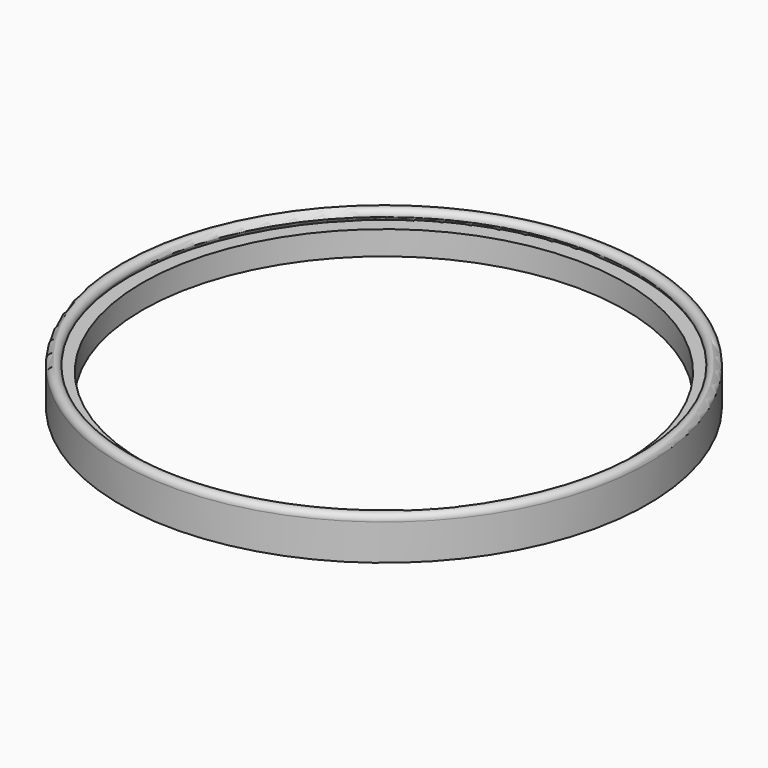
from build123d import *

# Parameters (mm, degrees)
F0_W = 8.2200646866
F0_H = 9.3895217869


# Not quite as in the source:
# - a feature names something its author has since deleted; it is built from what else it names


with BuildPart() as f1:
    # F0 (on Front) → F1 (revolve)
    with BuildSketch(Plane.XZ):
        with BuildLine():
            Line((0, 19), (0, 0))
            Line((0, 0), (0.6, 0))
            Line((0.6, 0), (0.6, 3.5557271383))
            Line((0.6, 3.5557271383), (11.9, 3.5557271383))
            Line((11.9, 3.5557271383), (11.9, 16.2557271383))
            Line((11.9, 16.2557271383), (3.2369840445, 16.2557271383))
            ThreePointArc((3.2369840445, 16.2557271383), (5.2521158412, 17.0766330758), (6.1823196963, 19.0437028519))
            Line((6.1823196963, 19.0437028519), (6.3827879741, 19.0437028519))
            ThreePointArc((6.3827879741, 19.0437028519), (3.1678853473, 22.4552809766), (0, 19))
        make_face()
        with Locations((6.2782712048, 9.8272700561)):
            Rectangle(F0_W, F0_H, mode=Mode.SUBTRACT)
    revolve(axis=Axis((139.7, 0, -5.7849194854), (0, 0, -1)))


solid = f1.part
